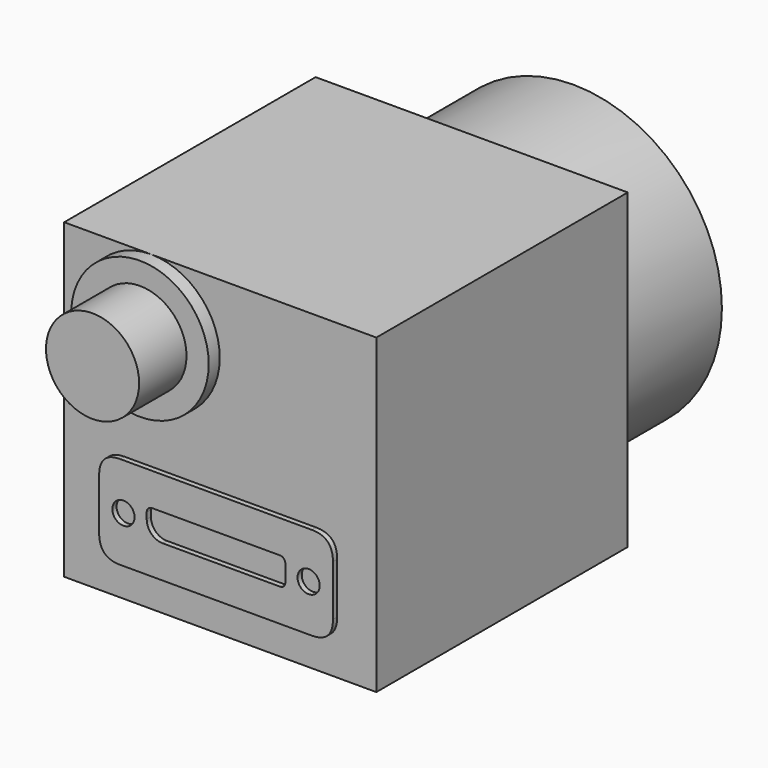
from build123d import *

# Parameters (mm, degrees)
F0_R        = 14.05
F1_DEPTH    = 12
F0_W        = 29.5
F0_H        = 29.5
F2_DEPTH    = 29.7
F3_DEPTH    = 29.7
F5_R        = 6.5
F5_R_2      = 4.4
F6_DEPTH    = 1.3
F7_DEPTH    = 6.9
F5_W        = 22.1
F5_H        = 8.8
F5_W_2      = 13.1
F5_H_2      = 2.6
F8_DEPTH    = 0.5
F9_T1_DEPTH = 5.5
F10_D       = 2.1
F10_DEPTH   = 6.901
F11_R       = 0.5
F12_R       = 1.5


# Not quite as in the source:
# - a fillet or chamfer that OpenCascade refuses, or shapes differently, is made with other operations: its cross-section is extruded or revolved along the edge and cut away or added


with BuildPart() as f1:
    # F0 (on Front) → F1 (new body)
    with BuildSketch(Plane.XZ):
        Circle(F0_R)
    extrude(amount=-F1_DEPTH)

    # F0 (on Front) → F2 (join)
    with BuildSketch(Plane.XZ):
        Rectangle(F0_W, F0_H)
        Circle(F0_R, mode=Mode.SUBTRACT)
    extrude(amount=F2_DEPTH)

    # F0 (on Front) → F3 (join)
    with BuildSketch(Plane.XZ):
        Circle(F0_R)
    extrude(amount=F3_DEPTH)

    # F5 (on offset) → F6 (join)
    with BuildSketch(Plane.XZ.offset(29.7)):
        with Locations((-6.55, 8.2499999553)):
            Circle(F5_R)
        with Locations((-6.55, 8.2499999553)):
            Circle(F5_R_2, mode=Mode.SUBTRACT)
    extrude(amount=F6_DEPTH)

    # F5 (on offset) → F7 (join)
    with BuildSketch(Plane.XZ.offset(29.7)):
        with Locations((-6.55, 8.2499999553)):
            Circle(F5_R_2)
    extrude(amount=F7_DEPTH)

    # F5 (on offset) → F8 (join)
    with BuildSketch(Plane.XZ.offset(29.7)):
        with Locations((-6.55, 8.2499999553)):
            Circle(F5_R)
        with Locations((-6.55, 8.2499999553)):
            Circle(F5_R_2, mode=Mode.SUBTRACT)
        with Locations((0, -7.3)):
            Rectangle(F5_W, F5_H)
        with Locations((0, -7.3)):
            Rectangle(F5_W_2, F5_H_2, mode=Mode.SUBTRACT)
    extrude(amount=F8_DEPTH)

    # F9: fillet of radius 2 on 4 edges, made by hand

    # F9_s2 → F9_t1 (cut)
    with BuildSketch(Plane.XZ.offset(29.7)):
        with BuildLine():
            add(Edge.make_bspline(
                [(-9.05, -2.9), (-11.05, -2.9), (-11.05, -4.9)],
                knots=[0, 0, 0, 1, 1, 1], degree=2, weights=[1, 1, 1]))
            Line((-11.05, -4.9), (-11.05, -2.9))
            Line((-11.05, -2.9), (-9.05, -2.9))
        make_face()
        with BuildLine():
            add(Edge.make_bspline(
                [(9.05, -2.9), (11.05, -2.9), (11.05, -4.9)],
                knots=[0, 0, 0, 1, 1, 1], degree=2, weights=[1, 1, 1]))
            Line((11.05, -4.9), (11.05, -2.9))
            Line((11.05, -2.9), (9.05, -2.9))
        make_face()
        with BuildLine():
            add(Edge.make_bspline(
                [(-9.05, -11.7), (-11.05, -11.7), (-11.05, -9.7)],
                knots=[0, 0, 0, 1, 1, 1], degree=2, weights=[1, 1, 1]))
            Line((-11.05, -9.7), (-11.05, -11.7))
            Line((-11.05, -11.7), (-9.05, -11.7))
        make_face()
        with BuildLine():
            add(Edge.make_bspline(
                [(11.05, -9.7), (11.05, -11.7), (9.05, -11.7)],
                knots=[0, 0, 0, 1, 1, 1], degree=2, weights=[1, 1, 1]))
            Line((9.05, -11.7), (11.05, -11.7))
            Line((11.05, -11.7), (11.05, -9.7))
        make_face()
    extrude(amount=F9_T1_DEPTH, mode=Mode.SUBTRACT)

    # F10 (through all, one way)
    with BuildSketch(Plane(origin=(0, -29.7, 0), x_dir=(1, 0, 0), z_dir=(0, 1, 0))):
        with Locations((-8.75, 7.3), (8.75, 7.3)):
            Circle(F10_D / 2)
    extrude(amount=-F10_DEPTH, mode=Mode.SUBTRACT)

    # F11
    f11_edges = [f1.edges().sort_by_distance(p)[0] for p in [
        (-6.55, -29.95, -6),
        (6.55, -29.95, -6),
        (6.55, -29.95, -8.6),
    ]]
    fillet(f11_edges, radius=F11_R)

    # F12
    f12_edges = [f1.edges().sort_by_distance(p)[0] for p in [
        (-6.55, -29.95, -8.6),
    ]]
    fillet(f12_edges, radius=F12_R)


solid = f1.part
